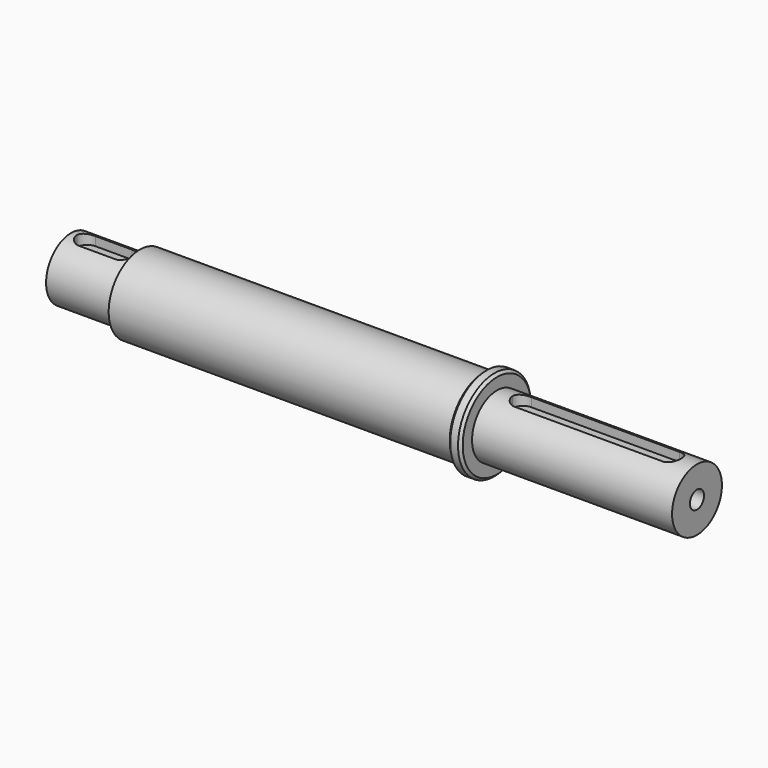
from build123d import *

# Parameters (mm, degrees)
F0_R      = 15
F1_DEPTH  = 164
F2_R      = 12
F3_DEPTH  = 77
F5_D      = 6.8
F5_DEPTH  = 30
F5_TIP    = 2.0429261047
F8_DEPTH  = 4.1
F9_R      = 17.5
F9_R_2    = 15
F10_DEPTH = 5
F11_SIZE  = 1
F12_R     = 15
F12_R_2   = 12
F13_DEPTH = 26.5
F14_D     = 6.8
F14_DEPTH = 20.75
F14_TIP   = 2.0429261047
F16_DEPTH = 4.1


# Not quite as in the source:
# - a feature names something its author has since deleted; it is built from what else it names


with BuildPart() as f1:
    # F0 (on Right) → F1 (new body)
    with BuildSketch(Plane.YZ):
        Circle(F0_R)
    extrude(amount=F1_DEPTH)

    # F2 (on face) → F3 (join)
    with BuildSketch(Plane.YZ.offset(164)):
        Circle(F2_R)
    extrude(amount=F3_DEPTH)

    # F5
    with Locations(Plane.YZ.offset(241)):
        with Locations((0, 0)):
            Hole(F5_D / 2, depth=F5_DEPTH)
            with Locations((0, 0, -(F5_DEPTH + F5_TIP / 2))):  # 118° drill point
                Cone(0, F5_D / 2, F5_TIP, mode=Mode.SUBTRACT)

    # F7 (on offset) → F8 (cut)
    with BuildSketch(Plane.XY.offset(12)):
        with BuildLine():
            ThreePointArc((170, 0), (171.1715728753, -2.8284271247), (174, -4))
            Line((174, -4), (231, -4))
            ThreePointArc((231, -4), (233.8284271247, -2.8284271247), (235, 0))
            ThreePointArc((235, 0), (233.8284271247, 2.8284271247), (231, 4))
            Line((231, 4), (174, 4))
            ThreePointArc((174, 4), (171.1715728753, 2.8284271247), (170, 0))
        make_face()
    extrude(amount=-F8_DEPTH, mode=Mode.SUBTRACT)

    # F9 (on face) → F10 (join)
    with BuildSketch(Plane.YZ.offset(164)):
        Circle(F9_R)
        Circle(F9_R_2, mode=Mode.SUBTRACT)
    extrude(amount=-F10_DEPTH)

    # F11
    f11_edges = [f1.edges().sort_by_distance(p)[0] for p in [
        (164, -17.5, 0),
        (159, -17.5, 0),
    ]]
    chamfer(f11_edges, length=F11_SIZE)

    # F12 (on face) → F13 (cut)
    with BuildSketch(Plane(origin=(0, 0, 0), x_dir=(0, -1, 0), z_dir=(-1, 0, 0))):
        Circle(F12_R)
        Circle(F12_R_2, mode=Mode.SUBTRACT)
    extrude(amount=-F13_DEPTH, mode=Mode.SUBTRACT)

    # F14
    with Locations(Plane(origin=(0, 0, 0), x_dir=(0, -1, 0), z_dir=(-1, 0, 0))):
        with Locations((0, 0)):
            Hole(F14_D / 2, depth=F14_DEPTH)
            with Locations((0, 0, -(F14_DEPTH + F14_TIP / 2))):  # 118° drill point
                Cone(0, F14_D / 2, F14_TIP, mode=Mode.SUBTRACT)

    # F15 (on offset) → F16 (cut)
    with BuildSketch(Plane.XY.offset(12)):
        with BuildLine():
            Line((6.25, -4), (20.25, -4))
            ThreePointArc((20.25, -4), (23.0784271247, -2.8284271247), (24.25, 0))
            ThreePointArc((24.25, 0), (23.0784271247, 2.8284271247), (20.25, 4))
            Line((20.25, 4), (6.25, 4))
            ThreePointArc((6.25, 4), (3.4215728753, 2.8284271247), (2.25, 0))
            ThreePointArc((2.25, 0), (3.4215728753, -2.8284271247), (6.25, -4))
        make_face()
    extrude(amount=-F16_DEPTH, mode=Mode.SUBTRACT)


solid = f1.part
